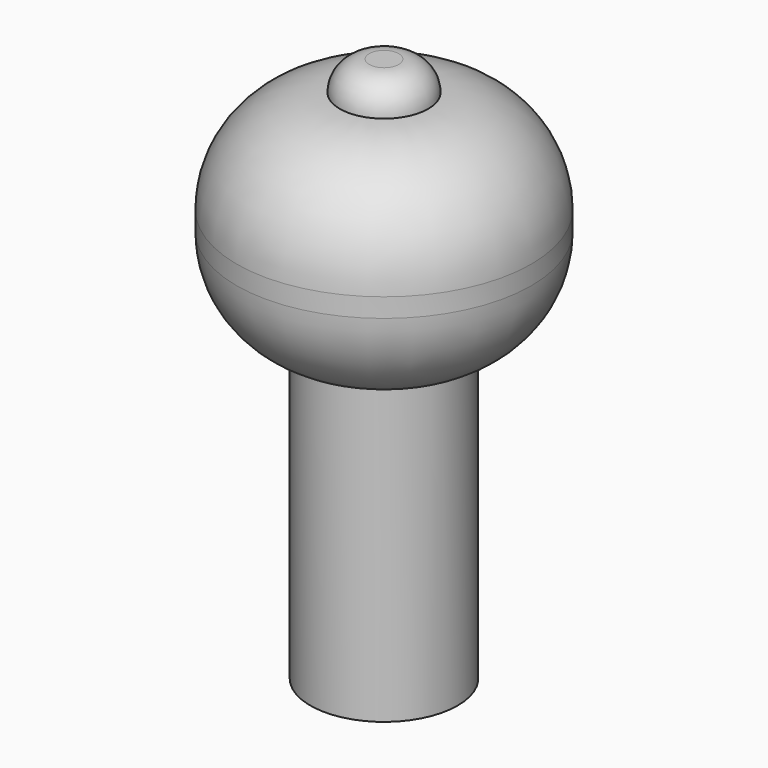
from build123d import *

# Parameters (mm, degrees)
F0_R     = 5
F1_DEPTH = 20
F2_R     = 10
F2_R_2   = 5
F3_DEPTH = 15
F5_DEPTH = 2
F6_R     = 1.99999


# Not quite as in the source:
# - a fillet or chamfer that OpenCascade refuses, or shapes differently, is made with other operations: its cross-section is extruded or revolved along the edge and cut away or added
# - a fillet or chamfer is up to 0.001 mm smaller than in the source, because OpenCascade refuses the exact size


with BuildPart() as f1:
    # F0 (on Top) → F1 (new body)
    with BuildSketch(Plane.XY):
        Circle(F0_R)
    extrude(amount=F1_DEPTH)

    # F2 (on face) → F3 (join)
    with BuildSketch(Plane.XY.offset(20)):
        Circle(F2_R)
        Circle(F2_R_2, mode=Mode.SUBTRACT)
        Circle(F2_R_2)
    extrude(amount=F3_DEPTH)

    # F4: fillet of radius 7 on 2 edges, made by hand

    # F4_s1 → F4_t2 (revolve, cut)
    with BuildSketch(Plane.XZ):
        with BuildLine():
            ThreePointArc((10, 28), (7.9497474683, 32.9497474683), (3, 35))
            Line((3, 35), (10, 35))
            Line((10, 35), (10, 28))
        make_face()
    revolve(axis=Axis((0, 0, 35), (0, 0, 1)), mode=Mode.SUBTRACT)

    # F4_s3 → F4_t4 (revolve, cut)
    with BuildSketch(Plane.XZ):
        with BuildLine():
            ThreePointArc((10, 26.7082039325), (8.6124860802, 22.5249037998), (5, 20))
            Line((5, 20), (10, 20))
            Line((10, 20), (10, 26.7082039325))
        make_face()
    revolve(axis=Axis((0, 0, 20), (0, 0, 1)), mode=Mode.SUBTRACT)

    # F5 (add): a face of the model
    f5_faces = [f1.faces().sort_by_distance(p)[0] for p in [
        (0, 0, 35),
    ]]
    extrude(f5_faces, amount=F5_DEPTH)

    # F6 (radius 2 in the source; OpenCascade refuses exactly that, so slightly less here)
    f6_edges = [f1.edges().sort_by_distance(p)[0] for p in [
        (-3, 0, 37),
    ]]
    fillet(f6_edges, radius=F6_R)


solid = f1.part
